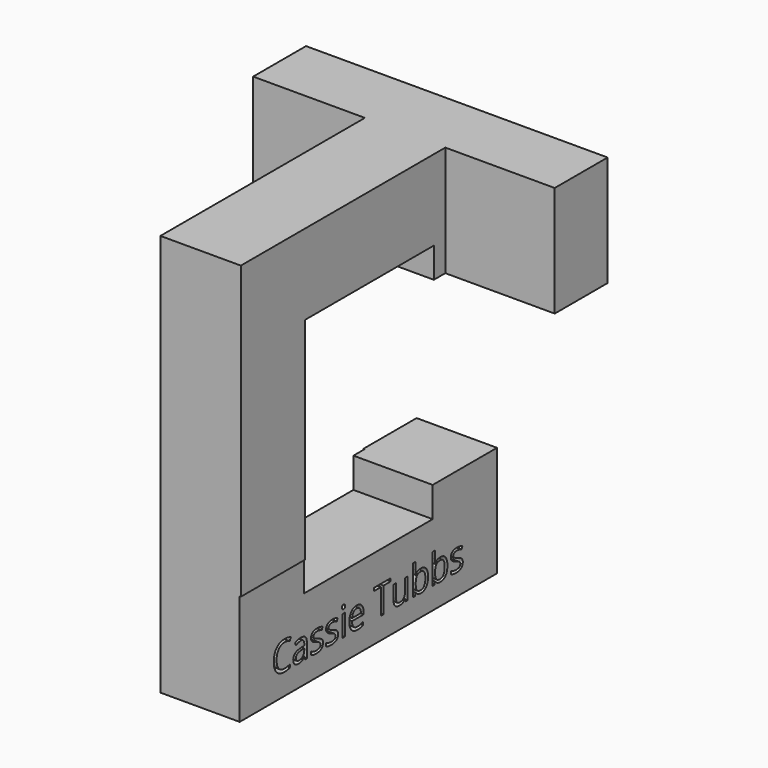
from build123d import *

# Parameters (mm, degrees)
F0_W         = 40
F0_H         = 40
F1_DEPTH     = 40
F5_DEPTH     = 40
F6_DEPTH     = 40
F7_DEPTH     = 40
F8_TEXT_SIZE = 3.9321116678
F9_DEPTH     = 5
F10_R        = 1
F11_DEPTH    = 4


# Not quite as in the source:
# - Text() gives the source's letters only with a copy of the font that has no kerning and outlines rounded to 1/6400 em; it was checked with that copy


with BuildPart() as f1:
    # F0 (on Top) → F1 (new body)
    with BuildSketch(Plane.XY):
        Rectangle(F0_W, F0_H)
    extrude(amount=-F1_DEPTH)

    # F2 (on face) → F5 (cut)
    with BuildSketch(Plane.XY):
        Polygon((-3.8847720716, -20), (-3.8847720716, 5.4262708873), (-15, 5.4262708873), (-15, 12.0000122), (15, 12.0000122), (15, 5.4262708873), (4.1152279284, 5.4262708873), (4.1152279284, -20), (20, -20), (20, 20), (-20, 20), (-20, -20), align=None)
    extrude(amount=-F5_DEPTH, mode=Mode.SUBTRACT)

    # F3 (on face) → F6 (cut)
    with BuildSketch(Plane.YZ.offset(20)):
        Polygon((20, 0), (12.0000122, 0), (12.0000122, -11), (4.0000122, -11), (4.0000122, -8), (-12, -8), (-12, -32), (4.0000122, -32), (4.0000122, -29), (12.0000122, -29), (12.0000122, -40), (20, -40), align=None)
    extrude(amount=-F6_DEPTH, mode=Mode.SUBTRACT)

    # F4 (on face) → F7 (cut)
    with BuildSketch(Plane.XZ.offset(20)):
        Polygon((-4, -32.0000122), (-4, -29), (-15.2172535012, -29), (-15.2172535012, -40), (-4, -40), align=None)
        Polygon((15.0087464988, -29), (4, -29), (4, -32.0000122), (4, -40), (15.0087464988, -40), align=None)
    extrude(amount=-F7_DEPTH, mode=Mode.SUBTRACT)

    # F8 (on face) → F9 (cut)
    with BuildSketch(Plane.YZ.offset(4)):
        with Locations((-16, -37.849189358)):
            Text('Cassie Tubbs', F8_TEXT_SIZE, font='Open Sans', text_align=(TextAlign.LEFT, TextAlign.BOTTOM))
    extrude(amount=-F9_DEPTH, mode=Mode.SUBTRACT)

    # F10 (on face) → F11 (cut)
    with BuildSketch(Plane(origin=(0, 0, -40), x_dir=(1, 0, 0), z_dir=(0, 0, -1))):
        with Locations((0.0288069821, 3.9999939)):
            Circle(F10_R)
    extrude(amount=-F11_DEPTH, mode=Mode.SUBTRACT)


solid = f1.part
